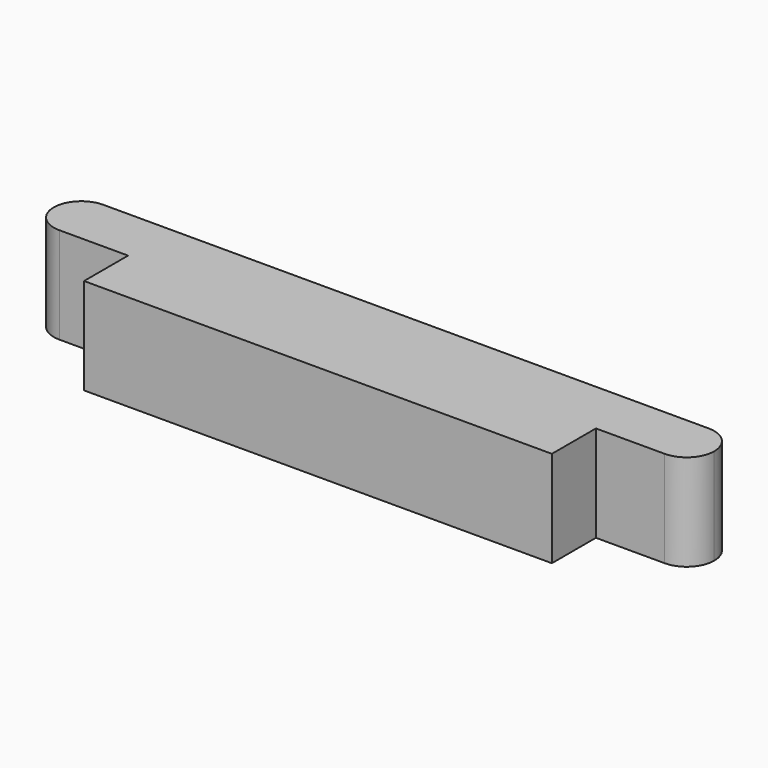
from build123d import *

# Parameters (mm, degrees)
F0_W     = 34
F0_H     = 4
F1_DEPTH = 7
F2_R     = 1.99999


# Not quite as in the source:
# - a fillet or chamfer is up to 0.001 mm smaller than in the source, because OpenCascade refuses the exact size


with BuildPart() as f1:
    # F0 (on Top) → F1 (new body)
    with BuildSketch(Plane.XY):
        Polygon((48, 0), (0, 0), (0, -4), (7, -4), (41, -4), (48, -4), align=None)
        with Locations((24, -6)):
            Rectangle(F0_W, F0_H)
    extrude(amount=F1_DEPTH)

    # F2 (radius 2 in the source; OpenCascade refuses exactly that, so slightly less here)
    f2_edges = [f1.edges().sort_by_distance(p)[0] for p in [
        (48, -4, 3.5),
        (48, 0, 3.5),
        (0, -4, 3.5),
        (0, 0, 3.5),
    ]]
    fillet(f2_edges, radius=F2_R)


solid = f1.part
